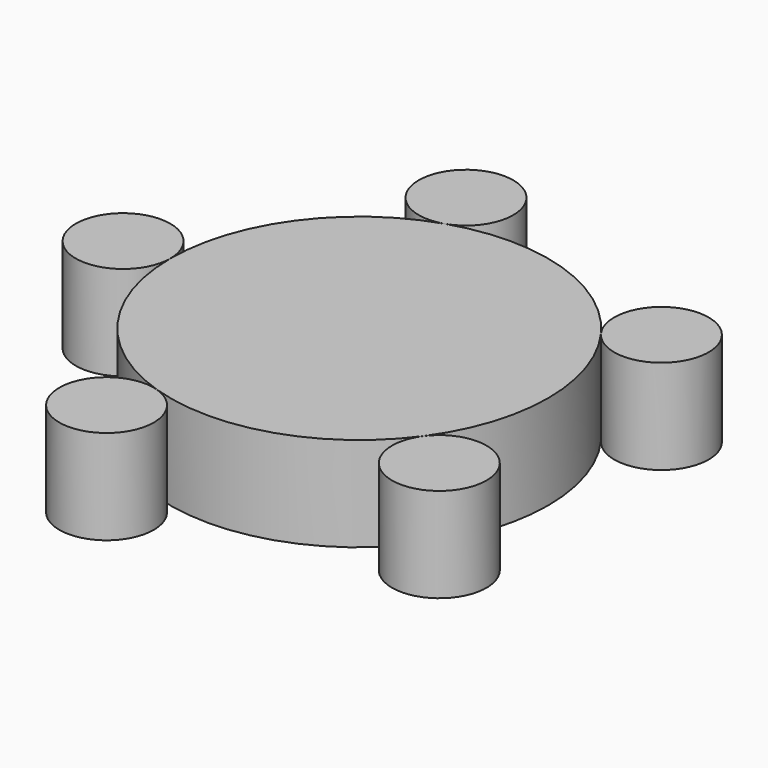
from build123d import *

# Parameters (mm, degrees)
F1_DEPTH = 25
F0_R     = 12.5
F2_DEPTH = 25
F3_COUNT = 5


with BuildPart() as f1:
    # F0 (on Top) → F1 (new body)
    with BuildSketch(Plane.XY):
        with BuildLine():
            ThreePointArc((-50, 0), (0, -50), (50, 0))
            ThreePointArc((50, 0), (0, 50), (-50, 0))
        make_face()
    extrude(amount=F1_DEPTH)


with BuildPart() as f2:
    # F0 (on Top) → F2 (new body)
    with BuildSketch(Plane.XY):
        with Locations((-62.5, 0)):
            Circle(F0_R)
    extrude(amount=F2_DEPTH)


with BuildPart() as f3_1:
    # F3: instance of F2
    add(f2.part.rotate(Axis((0, 0, 25), (0, 0, -1)), 1 * 360 / F3_COUNT))


with BuildPart() as f3_2:
    # F3: instance of F2
    add(f2.part.rotate(Axis((0, 0, 25), (0, 0, -1)), 2 * 360 / F3_COUNT))


with BuildPart() as f3_3:
    # F3: instance of F2
    add(f2.part.rotate(Axis((0, 0, 25), (0, 0, -1)), 3 * 360 / F3_COUNT))


with BuildPart() as f3_4:
    # F3: instance of F2
    add(f2.part.rotate(Axis((0, 0, 25), (0, 0, -1)), 4 * 360 / F3_COUNT))


solid = Compound([f1.part, f2.part, f3_1.part, f3_2.part, f3_3.part, f3_4.part])
